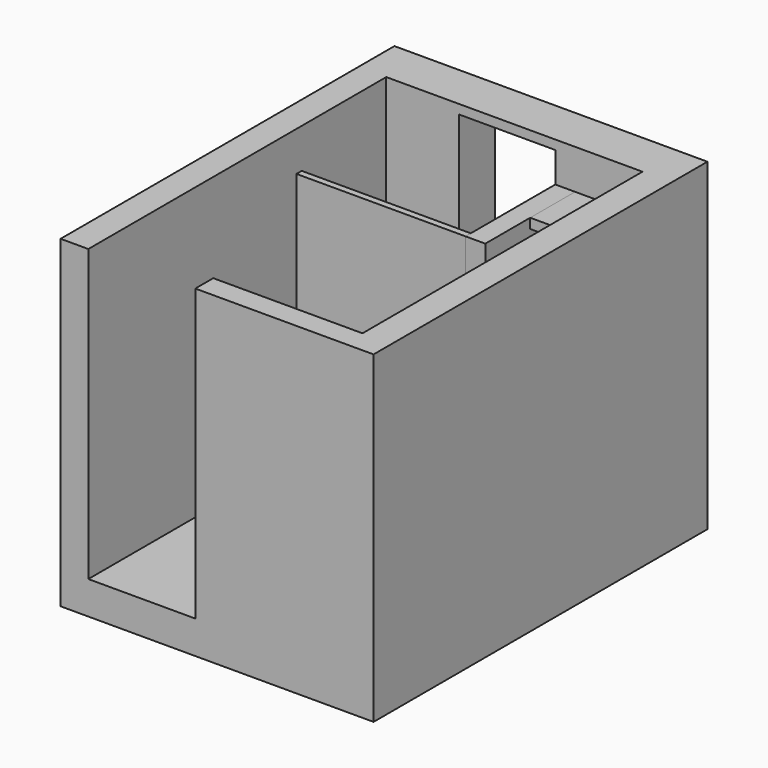
from build123d import *

# Parameters (mm, degrees)
F2_DEPTH  = 220
F3_W      = 73
F3_H      = 34
F4_DEPTH  = 92
F5_W      = 73
F5_H      = 34
F6_DEPTH  = 7
F7_W      = 237
F7_H      = 316
F8_DEPTH  = 25
F9_W      = 40
F9_H      = 85
F10_DEPTH = 10
F11_R     = 2.5
F12_DEPTH = 25
F13_DEPTH = 20
F15_DEPTH = 45
F16_W     = 65
F16_H     = 85
F17_DEPTH = 60
F18_W     = 47.9200673103
F18_H     = 65
F19_DEPTH = 10
F20_W     = 65
F20_H     = 56.4966313541
F21_DEPTH = 60
F22_R     = 6.0685644394
F23_DEPTH = 56.4966313541
F24_W     = 37.9200673103
F24_H     = 55
F25_DEPTH = 5
F27_DEPTH = 5
F29_DEPTH = 123
F30_W     = 45
F30_H     = 80
F31_DEPTH = 55
F32_DEPTH = 5
F34_DEPTH = 5
F35_DEPTH = 62
F37_W     = 51
F37_H     = 7.5
F38_DEPTH = 85
F39_W     = 51
F39_H     = 7.5
F40_DEPTH = 70.8
F41_W     = 51
F41_H     = 7.5
F42_DEPTH = 56.7
F43_W     = 51
F43_H     = 7.5
F44_DEPTH = 42.5


with BuildPart() as f2:
    # F1 (on Top) → F2 (new body)
    with BuildSketch(Plane.XY):
        Polygon((224, 406), (290, 406), (290, 141), (177, 141), (177, 124), (290, 124), (312, 124), (312, 406), (312, 440), (75, 440), (75, 406), (75, 141), (75, 124), (96, 124), (96, 222), (96, 406), (151, 406), align=None)
    extrude(amount=F2_DEPTH)

    # F3 (on face) → F4 (cut)
    with BuildSketch(Plane.XY.offset(220)):
        with Locations((187.5, 423)):
            Rectangle(F3_W, F3_H)
    extrude(amount=-F4_DEPTH, mode=Mode.SUBTRACT)

    # F5 (on face) → F6 (join)
    with BuildSketch(Plane.XY.offset(220)):
        with Locations((187.5, 423)):
            Rectangle(F5_W, F5_H)
    extrude(amount=-F6_DEPTH)

    # F7 (on face) → F8 (join)
    with BuildSketch(Plane(origin=(0, 0, 0), x_dir=(1, 0, 0), z_dir=(0, 0, -1))):
        with Locations((193.5, -282)):
            Rectangle(F7_W, F7_H)
    extrude(amount=F8_DEPTH)

    # F11 (on face) → F12 (cut)
    with BuildSketch(Plane.XY):
        with Locations((106, 366)):
            Circle(F11_R)
    extrude(amount=-F12_DEPTH, mode=Mode.SUBTRACT)

    # F26 (on face) → F27 (join)
    with BuildSketch(Plane.XY):
        Polygon((96, 326), (96, 321), (239, 321), (239, 406), (224, 406), (224, 326), align=None)
    extrude(amount=F27_DEPTH)

    # F28 (on face) → F29 (join, through all)
    with BuildSketch(Plane.XY.offset(5)):
        Polygon((239, 406), (224, 406), (224, 326), (224, 321), (239, 321), align=None)
    extrude(amount=F29_DEPTH)

    # F30 (on face) → F31 (join)
    with BuildSketch(Plane.XY):
        with Locations((201.5, 366)):
            Rectangle(F30_W, F30_H)
    extrude(amount=F31_DEPTH)

    # F32 (add, through all): a face of the model
    f32_faces = [f2.faces().sort_by_distance(p)[0] for p in [
        (201.5, 326, 30),
    ]]
    extrude(f32_faces, amount=F32_DEPTH)

    # F35 (add, through all): a face of the model
    f35_faces = [f2.faces().sort_by_distance(p)[0] for p in [
        (231.5, 363.5, 128),
    ]]
    extrude(f35_faces, amount=F35_DEPTH)


with BuildPart() as f10:
    # F9 (on face) → F10 (new body)
    with BuildSketch(Plane(origin=(290, 0, 0), x_dir=(0, -1, 0), z_dir=(-1, 0, 0))):
        with Locations((-258, 42.5)):
            Rectangle(F9_W, F9_H)
    extrude(amount=F10_DEPTH)

    # F9 (on face) → F13 (join)
    with BuildSketch(Plane(origin=(290, 0, 0), x_dir=(0, -1, 0), z_dir=(-1, 0, 0))):
        with Locations((-258, 42.5)):
            Rectangle(F9_W, F9_H)
    extrude(amount=F13_DEPTH)

    # F14 (on face) → F15 (join)
    with BuildSketch(Plane(origin=(270, 0, 0), x_dir=(0, -1, 0), z_dir=(-1, 0, 0))):
        Polygon((-238, 0), (-238, 42.5), (-258, 42.5), (-278, 42.5), (-278, 0), align=None)
    extrude(amount=F15_DEPTH)


with BuildPart() as f17:
    # F16 (on face) → F17 (new body)
    with BuildSketch(Plane(origin=(290, 0, 0), x_dir=(0, -1, 0), z_dir=(-1, 0, 0))):
        with Locations((-191, 42.5)):
            Rectangle(F16_W, F16_H)
    extrude(amount=F17_DEPTH)

    # F18 (on face) → F19 (cut)
    with BuildSketch(Plane.XY.offset(85)):
        with Locations((253.9600336552, 191)):
            Rectangle(F18_W, F18_H)
    extrude(amount=-F19_DEPTH, mode=Mode.SUBTRACT)

    # F20 (on face) → F21 (cut, through all)
    with BuildSketch(Plane(origin=(230, 0, 0), x_dir=(0, -1, 0), z_dir=(-1, 0, 0))):
        with Locations((-191, 28.248315677)):
            Rectangle(F20_W, F20_H)
    extrude(amount=-F21_DEPTH, mode=Mode.SUBTRACT)

    # F22 (on face) → F23 (join, through all)
    with BuildSketch(Plane(origin=(0, 0, 56.4966313541), x_dir=(1, 0, 0), z_dir=(0, 0, -1))):
        with Locations((260.0000000006, -191)):
            Circle(F22_R)
    extrude(amount=F23_DEPTH)

    # F24 (on face) → F25 (cut)
    with BuildSketch(Plane.XY.offset(75)):
        with Locations((253.9600336552, 191)):
            Rectangle(F24_W, F24_H)
    extrude(amount=-F25_DEPTH, mode=Mode.SUBTRACT)


with BuildPart() as f34:
    # F33 (on face) → F34 (new body, through all)
    with BuildSketch(Plane.XZ.offset(-321)):
        Polygon((179, 5), (179, 55), (224, 55), (224, 190), (96, 190), (96, 5), align=None)
    extrude(amount=-F34_DEPTH)


with BuildPart() as f38:
    # F37 (on face) → F38 (new body)
    with BuildSketch(Plane.XZ.offset(-406)):
        with Locations((264.5, 43.75)):
            Rectangle(F37_W, F37_H)
    extrude(amount=F38_DEPTH)


with BuildPart() as f40:
    # F39 (on face) → F40 (new body)
    with BuildSketch(Plane.XZ.offset(-406)):
        with Locations((264.5, 91.25)):
            Rectangle(F39_W, F39_H)
    extrude(amount=F40_DEPTH)


with BuildPart() as f42:
    # F41 (on face) → F42 (new body)
    with BuildSketch(Plane.XZ.offset(-406)):
        with Locations((264.5, 138.75)):
            Rectangle(F41_W, F41_H)
    extrude(amount=F42_DEPTH)


with BuildPart() as f44:
    # F43 (on face) → F44 (new body)
    with BuildSketch(Plane.XZ.offset(-406)):
        with Locations((264.5, 186.25)):
            Rectangle(F43_W, F43_H)
    extrude(amount=F44_DEPTH)


solid = Compound([f2.part, f10.part, f17.part, f34.part, f38.part, f40.part, f42.part, f44.part])
